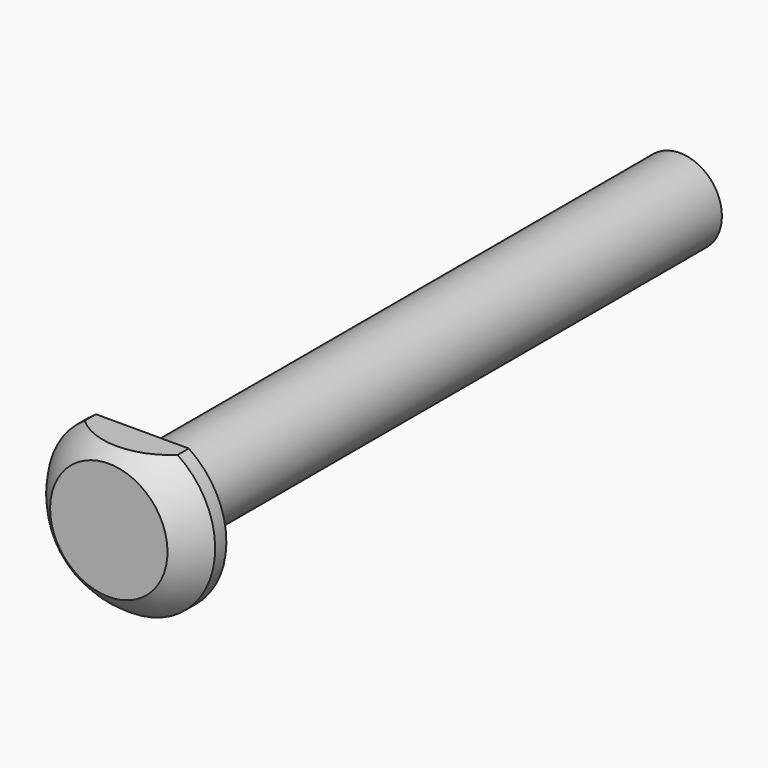
from build123d import *

# Parameters (mm, degrees)
F0_R     = 4.7625
F1_DEPTH = 76.2
F2_R     = 9.525
F2_R_2   = 4.7625
F3_DEPTH = 1.5875
F7_DEPTH = 25.4


# Not quite as in the source:
# - a length typed as a fraction of an inch, garbled in the dataset ("3 / 203.2 mm" for 3/8 in), is restored


with BuildPart() as f1:
    # F0 (on Front) → F1 (new body)
    with BuildSketch(Plane.XZ):
        with Locations((0, 5.2942009643)):
            Circle(F0_R)
    extrude(amount=F1_DEPTH)

    # F2 (on face) → F3 (join)
    with BuildSketch(Plane.XZ.offset(76.2)):
        with Locations((0, 5.2942009643)):
            Circle(F2_R)
        with Locations((0, 5.2942009643)):
            Circle(F2_R_2, mode=Mode.SUBTRACT)
        with Locations((0, 5.2942009643)):
            Circle(F2_R_2)
    extrude(amount=F3_DEPTH)

    # F4 (on Right) → F5 (revolve)
    with BuildSketch(Plane.YZ):
        with BuildLine():
            ThreePointArc((-80.9625, -1.3615326297), (-79.514423226, -2.9504452476), (-77.7875, -4.2307990357))
            Line((-77.7875, -4.2307990357), (-77.7875, 5.2942009643))
            Line((-77.7875, 5.2942009643), (-80.9625, 5.2942009643))
            Line((-80.9625, 5.2942009643), (-80.9625, -1.3615326297))
        make_face()
    revolve(axis=Axis((0, -79.375, 5.2942009643), (0, 1, 0)))

    # F6 (on face) → F7 (cut)
    with BuildSketch(Plane(origin=(0, -76.2, 0), x_dir=(-1, 0, 0), z_dir=(0, 1, 0))):
        with BuildLine():
            Line((0, 13.2317009643), (5.2651418547, 13.2317009643))
            ThreePointArc((5.2651418547, 13.2317009643), (0, 14.8192009643), (-5.2651418547, 13.2317009643))
            Line((-5.2651418547, 13.2317009643), (0, 13.2317009643))
        make_face()
    extrude(amount=-F7_DEPTH, mode=Mode.SUBTRACT)


solid = f1.part
